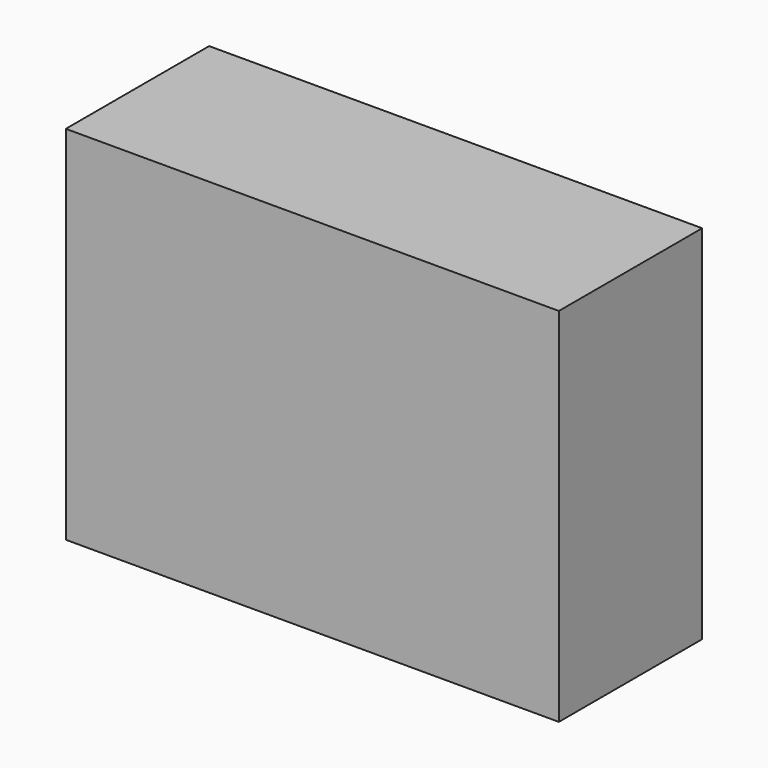
from build123d import *

# Parameters (mm, degrees)
F1_W     = 68.8026621938
F1_H     = 50.4858903587
F2_DEPTH = 25


# Not quite as in the source:
# - a feature of the source that left no trace in its solid (it failed there, or was rolled back) is left out


with BuildPart() as f2:
    # F1 (on Front) → F2 (new body)
    with BuildSketch(Plane.XZ):
        with Locations((-75.7120884955, 25.2429451793)):
            Rectangle(F1_W, F1_H)
    extrude(amount=F2_DEPTH)


solid = f2.part
